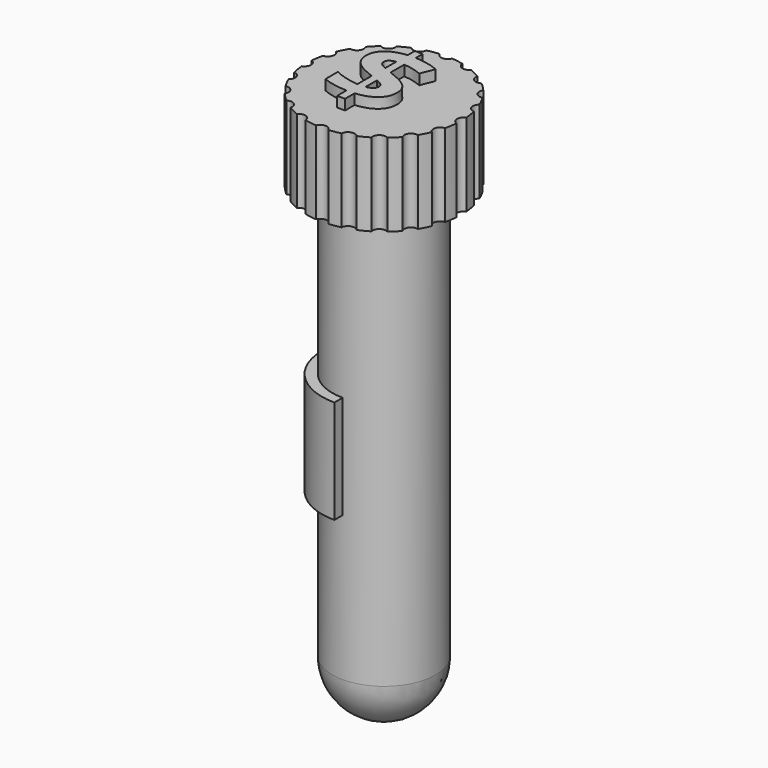
from build123d import *

# Parameters (mm, degrees)
F0_R         = 6.35
F1_DEPTH     = 50.8
F4_R         = 6.35
F5_DEPTH     = 10.16
F8_DEPTH     = 12.7
F9_TEXT_SIZE = 14.5962500634
F10_DEPTH    = 1.27


# Not quite as in the source:
# - Text() gives the source's letters only with a copy of the font that has no kerning and outlines rounded to 1/6400 em; it was checked with that copy


with BuildPart() as f1:
    # F0 (on Top) → F1 (new body)
    with BuildSketch(Plane.XY):
        Circle(F0_R)
    extrude(amount=-F1_DEPTH)

    # F2 (on face) → F3 (revolve)
    with BuildSketch(Plane(origin=(0, 0, -50.8), x_dir=(1, 0, 0), z_dir=(0, 0, -1))):
        with BuildLine():
            Line((0, 6.35), (0, -6.35))
            ThreePointArc((0, -6.35), (6.35, 0), (0, 6.35))
        make_face()
    revolve(axis=Axis((0, 0, -50.8), (0, 1, 0)))

    # F7 (on offset) → F8 (join)
    with BuildSketch(Plane.XY.offset(-20.32)):
        with BuildLine():
            Line((0, -7.62), (0, 7.62))
            ThreePointArc((0, 7.62), (-7.62, 0), (0, -7.62))
        make_face()
    extrude(amount=-F8_DEPTH)


with BuildPart() as f5:
    # F4 (on face) → F5 (new body)
    with BuildSketch(Plane.XY):
        with BuildLine():
            ThreePointArc((9.4944710753, -0.762), (8.9759289865, 0), (9.4944710753, 0.762))
            ThreePointArc((9.4944710753, 0.762), (9.4077314442, 1.4900382795), (9.2652495347, 2.2092478495))
            ThreePointArc((9.2652495347, 2.2092478495), (8.5366157524, 2.7737145971), (8.7943076352, 3.6586579803))
            ThreePointArc((8.7943076352, 3.6586579803), (8.4868371429, 4.32425951), (8.1290808148, 4.9642391267))
            ThreePointArc((8.1290808148, 4.9642391267), (7.2616790904, 5.2759186839), (7.2332960903, 6.1971810261))
            ThreePointArc((7.2332960903, 6.1971810261), (6.7351920908, 6.7351920908), (6.1971810261, 7.2332960903))
            ThreePointArc((6.1971810261, 7.2332960903), (5.2759186839, 7.2616790904), (4.9642391267, 8.1290808148))
            ThreePointArc((4.9642391267, 8.1290808148), (4.32425951, 8.4868371429), (3.6586579803, 8.7943076352))
            ThreePointArc((3.6586579803, 8.7943076352), (2.7737145971, 8.5366157524), (2.2092478495, 9.2652495347))
            ThreePointArc((2.2092478495, 9.2652495347), (1.4900382795, 9.4077314442), (0.762, 9.4944710753))
            ThreePointArc((0.762, 9.4944710753), (0, 8.9759289865), (-0.762, 9.4944710753))
            ThreePointArc((-0.762, 9.4944710753), (-1.4900382795, 9.4077314442), (-2.2092478495, 9.2652495347))
            ThreePointArc((-2.2092478495, 9.2652495347), (-2.7737145971, 8.5366157524), (-3.6586579803, 8.7943076352))
            ThreePointArc((-3.6586579803, 8.7943076352), (-4.32425951, 8.4868371429), (-4.9642391267, 8.1290808148))
            ThreePointArc((-4.9642391267, 8.1290808148), (-5.2759186839, 7.2616790904), (-6.1971810261, 7.2332960903))
            ThreePointArc((-6.1971810261, 7.2332960903), (-6.7351920908, 6.7351920908), (-7.2332960903, 6.1971810261))
            ThreePointArc((-7.2332960903, 6.1971810261), (-7.2616790904, 5.2759186839), (-8.1290808148, 4.9642391267))
            ThreePointArc((-8.1290808148, 4.9642391267), (-8.4868371429, 4.32425951), (-8.7943076352, 3.6586579803))
            ThreePointArc((-8.7943076352, 3.6586579803), (-8.5366157524, 2.7737145971), (-9.2652495347, 2.2092478495))
            ThreePointArc((-9.2652495347, 2.2092478495), (-9.4077314442, 1.4900382795), (-9.4944710753, 0.762))
            ThreePointArc((-9.4944710753, 0.762), (-8.9759289865, 0), (-9.4944710753, -0.762))
            ThreePointArc((-9.4944710753, -0.762), (-9.4077314442, -1.4900382795), (-9.2652495347, -2.2092478495))
            ThreePointArc((-9.2652495347, -2.2092478495), (-8.5366157524, -2.7737145971), (-8.7943076352, -3.6586579803))
            ThreePointArc((-8.7943076352, -3.6586579803), (-8.4868371429, -4.32425951), (-8.1290808148, -4.9642391267))
            ThreePointArc((-8.1290808148, -4.9642391267), (-7.2616790904, -5.2759186839), (-7.2332960903, -6.1971810261))
            ThreePointArc((-7.2332960903, -6.1971810261), (-6.7351920908, -6.7351920908), (-6.1971810261, -7.2332960903))
            ThreePointArc((-6.1971810261, -7.2332960903), (-5.2759186839, -7.2616790904), (-4.9642391267, -8.1290808148))
            ThreePointArc((-4.9642391267, -8.1290808148), (-4.32425951, -8.4868371429), (-3.6586579803, -8.7943076352))
            ThreePointArc((-3.6586579803, -8.7943076352), (-2.7737145971, -8.5366157524), (-2.2092478495, -9.2652495347))
            ThreePointArc((-2.2092478495, -9.2652495347), (-1.4900382795, -9.4077314442), (-0.762, -9.4944710753))
            ThreePointArc((-0.762, -9.4944710753), (0, -8.9759289865), (0.762, -9.4944710753))
            ThreePointArc((0.762, -9.4944710753), (1.4900382795, -9.4077314442), (2.2092478495, -9.2652495347))
            ThreePointArc((2.2092478495, -9.2652495347), (2.7737145971, -8.5366157524), (3.6586579803, -8.7943076352))
            ThreePointArc((3.6586579803, -8.7943076352), (4.32425951, -8.4868371429), (4.9642391267, -8.1290808148))
            ThreePointArc((4.9642391267, -8.1290808148), (5.2759186839, -7.2616790904), (6.1971810261, -7.2332960903))
            ThreePointArc((6.1971810261, -7.2332960903), (6.7351920908, -6.7351920908), (7.2332960903, -6.1971810261))
            ThreePointArc((7.2332960903, -6.1971810261), (7.2616790904, -5.2759186839), (8.1290808148, -4.9642391267))
            ThreePointArc((8.1290808148, -4.9642391267), (8.4868371429, -4.32425951), (8.7943076352, -3.6586579803))
            ThreePointArc((8.7943076352, -3.6586579803), (8.5366157524, -2.7737145971), (9.2652495347, -2.2092478495))
            ThreePointArc((9.2652495347, -2.2092478495), (9.4077314442, -1.4900382795), (9.4944710753, -0.762))
        make_face()
        Circle(F4_R, mode=Mode.SUBTRACT)
        Circle(F4_R)
    extrude(amount=F5_DEPTH)

    # F9 (on face) → F10 (join)
    with BuildSketch(Plane.XY.offset(10.16)):
        with Locations((-5.1719741896, -4.5003881678)):
            Text('$', F9_TEXT_SIZE, font='Open Sans', font_style=FontStyle.BOLD, text_align=(TextAlign.LEFT, TextAlign.BOTTOM))
    extrude(amount=F10_DEPTH)


solid = Compound([f1.part, f5.part])
